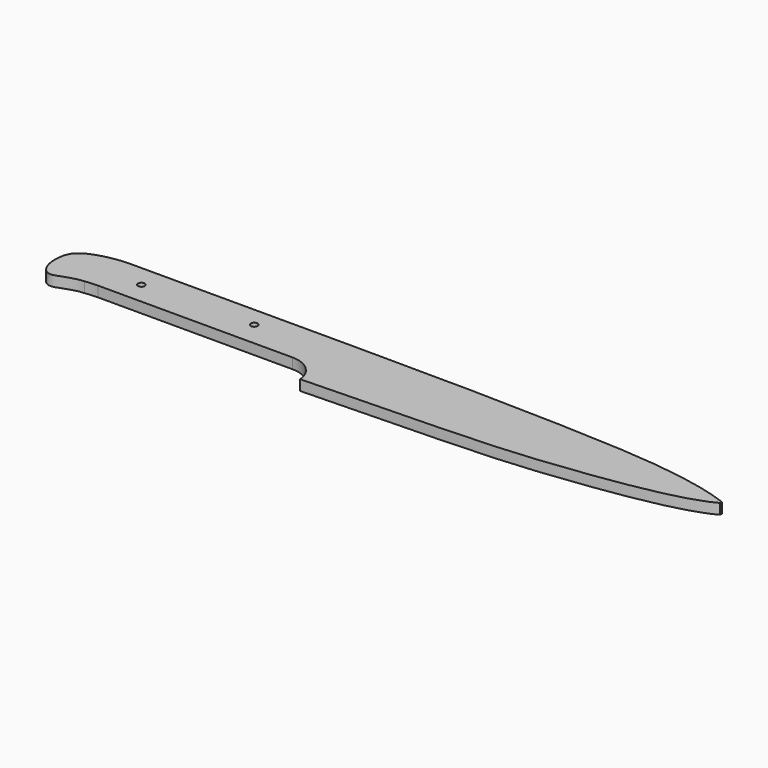
from build123d import *

# Parameters (mm, degrees)
F0_R     = 1.5875
F1_DEPTH = 4.7625


with BuildPart() as f1:
    # F0 (on Top) → F1 (new body)
    with BuildSketch(Plane.XY):
        with BuildLine():
            add(Edge.make_bspline(
                [(-25.4000339955, 19.0499999844), (11.0659803484, 19.0499999844), (75.6404907204, 18.3951374474), (131.6233865179, 14.5919578775), (151.4037655455, 7.2832109724)],
                knots=[0, 0, 0, 0, 0.5432073477, 0.9924282823, 0.9924282823, 0.9924282823, 0.9924282823], degree=3))
            Line((-25.4000339955, 19.0499999844), (-127, 19.0499999844))
            add(Edge.make_bspline(
                [(-132.8572214313, -1.7011073168), (-138.7224568365, -1.9098253759), (-146.5869393979, -7.9306938244), (-151.6875511275, 0.0750696788), (-151.8479933658, 7.2472530677), (-149.7515385788, 14.6964316511), (-136.3808090157, 18.8981087489), (-129.8206844988, 19.0301054596), (-127, 19.0499999844)],
                knots=[0, 0, 0, 0, 0.2045504807, 0.3449061653, 0.4915899731, 0.6341965753, 0.8315420062, 1, 1, 1, 1], degree=3))
            ThreePointArc((-132.8572214313, -1.7011073168), (-129.9365326669, -1.3779224016), (-127, -1.27))
            Line((-127, -1.27), (-38.1, -1.27))
            ThreePointArc((-38.1, -1.27), (-29.5805810057, -4.5514279214), (-25.4636595487, -12.7))
            add(Edge.make_bspline(
                [(-25.4636595487, -12.7), (48.6882164823, -10.6703078891), (71.671615255, -10.5113328002), (140.4678429521, -0.2739958712), (151.4037655455, 6.2728745575)],
                knots=[0, 0, 0, 0, 0.5771160301, 0.986879266, 0.986879266, 0.986879266, 0.986879266], degree=3))
            Line((151.4037655455, 6.2728745575), (151.4037655455, 7.2832109724))
        make_face()
        with Locations((-115.3946487784, 8.8899999844)):
            Circle(F0_R, mode=Mode.SUBTRACT)
        with Locations((-64.5946487784, 9.931572713)):
            Circle(F0_R, mode=Mode.SUBTRACT)
    extrude(amount=F1_DEPTH)


solid = f1.part
